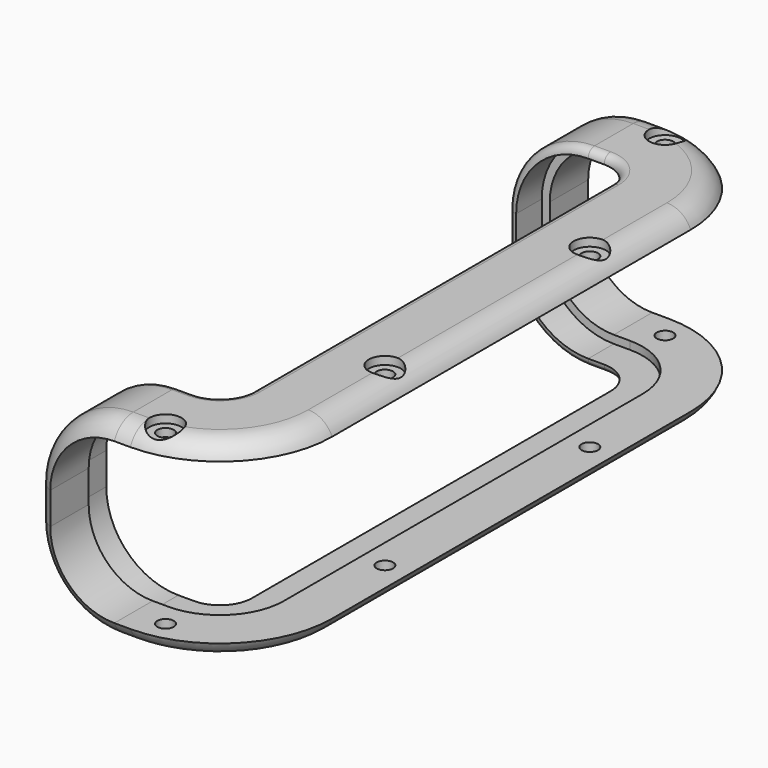
from build123d import *

# Parameters (mm, degrees)
F1_DEPTH      = 133.35
F2_R          = 12.7
F3_R          = 15.875
F4_R          = 22.225
F6_DEPTH      = 38.101
F8_DEPTH      = 6.35
F8_DEPTH_BACK = 107.95
F9_R          = 12.7
F10_T1_DEPTH  = 6.35
F10_T3_DEPTH  = 3.175
F10_T5_DEPTH  = 88.9
F10_T8_ANGLE  = 90
F10_T10_ANGLE = 90
F10_T12_ANGLE = 90
F10_T14_ANGLE = 90
F10_T16_ANGLE = 90
F10_T18_ANGLE = 90
F10_T20_ANGLE = 90
F10_T22_ANGLE = 90
F11_R         = 1.58749
F13_D         = 3.2639
F14_R         = 3.175
F15_DEPTH     = 1.5875


# Not quite as in the source:
# - a fillet or chamfer that OpenCascade refuses, or shapes differently, is made with other operations: its cross-section is extruded or revolved along the edge and cut away or added
# - a fillet or chamfer is up to 0.001 mm smaller than in the source, because OpenCascade refuses the exact size


with BuildPart() as f1:
    # F0 (on Front) → F1 (new body)
    with BuildSketch(Plane.XZ):
        Polygon((38.1, 0), (0, 0), (0, 31.75), (38.1, 31.75), (38.1, 34.925), (-3.175, 34.925), (-3.175, -3.175), (38.1, -3.175), align=None)
    extrude(amount=F1_DEPTH)

    # F2
    f2_edges = [f1.edges().sort_by_distance(p)[0] for p in [
        (0, -66.675, 0),
        (0, -66.675, 31.75),
    ]]
    fillet(f2_edges, radius=F2_R)

    # F3
    f3_edges = [f1.edges().sort_by_distance(p)[0] for p in [
        (-3.175, -66.675, -3.175),
        (-3.175, -66.675, 34.925),
    ]]
    fillet(f3_edges, radius=F3_R)

    # F4
    f4_edges = [f1.edges().sort_by_distance(p)[0] for p in [
        (38.1, -133.35, 33.3375),
        (38.1, -133.35, -1.5875),
        (38.1, 0, 33.3375),
        (38.1, 0, -1.5875),
    ]]
    fillet(f4_edges, radius=F4_R)

    # F5 (on face) → F6 (cut, through all)
    with BuildSketch(Plane.XY.offset(34.925)):
        with BuildLine():
            Line((-3.175, -117.475), (15.875, -117.475))
            ThreePointArc((15.875, -117.475), (20.3651280605, -115.6151280605), (22.225, -111.125))
            Line((22.225, -111.125), (22.225, -22.225))
            ThreePointArc((22.225, -22.225), (20.3651280605, -17.7348719395), (15.875, -15.875))
            Line((15.875, -15.875), (-3.175, -15.875))
            Line((-3.175, -15.875), (-3.175, -117.475))
        make_face()
    extrude(amount=-F6_DEPTH, mode=Mode.SUBTRACT)

    # F7 (on face) → F8 (cut, two sides)
    with BuildSketch(Plane(origin=(0, -117.475, 0), x_dir=(-1, 0, 0), z_dir=(0, 1, 0))) as f8_sk:
        with BuildLine():
            Line((-28.575, -1.5875), (-12.7, -1.5875))
            ThreePointArc((-12.7, -1.5875), (-2.5972118638, 2.5972118638), (1.5875, 12.7))
            Line((1.5875, 12.7), (1.5875, 19.05))
            ThreePointArc((1.5875, 19.05), (-2.5972118638, 29.1527881362), (-12.7, 33.3375))
            Line((-12.7, 33.3375), (-28.575, 33.3375))
            Line((-28.575, 33.3375), (-28.575, -1.5875))
        make_face()
    extrude(amount=-F8_DEPTH, mode=Mode.SUBTRACT)
    extrude(f8_sk.sketch, amount=F8_DEPTH_BACK, mode=Mode.SUBTRACT)

    # F9
    f9_edges = [f1.edges().sort_by_distance(p)[0] for p in [
        (28.575, -123.825, -0.79375),
        (28.575, -123.825, 32.54375),
        (28.575, -9.525, 32.54375),
        (28.575, -9.525, -0.79375),
    ]]
    fillet(f9_edges, radius=F9_R)

    # F10: fillet of radius 5.08 on 1 edges, made by hand

    # F10_s2 → F10_t1 (cut)
    with BuildSketch(Plane.XY.offset(12.7)):
        with BuildLine():
            ThreePointArc((0, -133.35), (-2.3071134838, -131.4805202921), (-3.175, -128.6407139607))
            Line((-3.175, -128.6407139607), (-3.175, -133.35))
            Line((-3.175, -133.35), (0, -133.35))
        make_face()
        with BuildLine():
            ThreePointArc((0, 0), (-2.3071134838, -1.8694797079), (-3.175, -4.7092860393))
            Line((-3.175, -4.7092860393), (-3.175, 0))
            Line((-3.175, 0), (0, 0))
        make_face()
    extrude(amount=F10_T1_DEPTH, mode=Mode.SUBTRACT)

    # F10_s4 → F10_t3 (cut)
    with BuildSketch(Plane.YZ.offset(12.7)):
        with BuildLine():
            ThreePointArc((-133.35, 31.75), (-131.4805202921, 34.0571134838), (-128.6407139607, 34.925))
            Line((-128.6407139607, 34.925), (-133.35, 34.925))
            Line((-133.35, 34.925), (-133.35, 31.75))
        make_face()
        with BuildLine():
            ThreePointArc((0, 31.75), (-1.8694797079, 34.0571134838), (-4.7092860393, 34.925))
            Line((-4.7092860393, 34.925), (0, 34.925))
            Line((0, 34.925), (0, 31.75))
        make_face()
        with BuildLine():
            ThreePointArc((0, 0), (-1.8694797079, -2.3071134838), (-4.7092860393, -3.175))
            Line((-4.7092860393, -3.175), (0, -3.175))
            Line((0, -3.175), (0, 0))
        make_face()
        with BuildLine():
            ThreePointArc((-133.35, 0), (-131.4805202921, -2.3071134838), (-128.6407139607, -3.175))
            Line((-128.6407139607, -3.175), (-133.35, -3.175))
            Line((-133.35, -3.175), (-133.35, 0))
        make_face()
    extrude(amount=F10_T3_DEPTH, mode=Mode.SUBTRACT)

    # F10_s6 → F10_t5 (cut)
    with BuildSketch(Plane.XZ.offset(22.225)):
        with BuildLine():
            ThreePointArc((33.3907139607, 34.925), (36.2305202921, 34.0571134838), (38.1, 31.75))
            Line((38.1, 31.75), (38.1, 34.925))
            Line((38.1, 34.925), (33.3907139607, 34.925))
        make_face()
        with BuildLine():
            ThreePointArc((38.1, 0), (36.2305202921, -2.3071134838), (33.3907139607, -3.175))
            Line((33.3907139607, -3.175), (38.1, -3.175))
            Line((38.1, -3.175), (38.1, 0))
        make_face()
    extrude(amount=F10_T5_DEPTH, mode=Mode.SUBTRACT)

    # F10_s7 → F10_t8 (revolve, cut)
    with BuildSketch(Plane.XY.offset(19.05)):
        with BuildLine():
            ThreePointArc((0, -133.35), (-2.3071134838, -131.4805202921), (-3.175, -128.6407139607))
            Line((-3.175, -128.6407139607), (-3.175, -133.35))
            Line((-3.175, -133.35), (0, -133.35))
        make_face()
    revolve(axis=Axis((12.7, -133.35, 19.05), (0, 1, 0)), revolution_arc=F10_T8_ANGLE, mode=Mode.SUBTRACT)

    # F10_s9 → F10_t10 (revolve, cut)
    with BuildSketch(Plane.XZ.offset(111.125)):
        with BuildLine():
            ThreePointArc((33.3907139607, 34.925), (36.2305202921, 34.0571134838), (38.1, 31.75))
            Line((38.1, 31.75), (38.1, 34.925))
            Line((38.1, 34.925), (33.3907139607, 34.925))
        make_face()
    revolve(axis=Axis((15.875, -111.125, 34.925), (0, 0, -1)), revolution_arc=F10_T10_ANGLE, mode=Mode.SUBTRACT)

    # F10_s11 → F10_t12 (revolve, cut)
    with BuildSketch(Plane.YZ.offset(15.875)):
        with BuildLine():
            ThreePointArc((-4.7092860393, 34.925), (-1.8694797079, 34.0571134838), (0, 31.75))
            Line((0, 31.75), (0, 34.925))
            Line((0, 34.925), (-4.7092860393, 34.925))
        make_face()
    revolve(axis=Axis((15.875, -22.225, 34.925), (0, 0, -1)), revolution_arc=F10_T12_ANGLE, mode=Mode.SUBTRACT)

    # F10_s13 → F10_t14 (revolve, cut)
    with BuildSketch(Plane.XY.offset(19.05)):
        with BuildLine():
            ThreePointArc((0, 0), (-2.3071134838, -1.8694797079), (-3.175, -4.7092860393))
            Line((-3.175, -4.7092860393), (-3.175, 0))
            Line((-3.175, 0), (0, 0))
        make_face()
    revolve(axis=Axis((12.7, 0, 19.05), (0, 1, 0)), revolution_arc=F10_T14_ANGLE, mode=Mode.SUBTRACT)

    # F10_s15 → F10_t16 (revolve, cut)
    with BuildSketch(Plane.YZ.offset(12.7)):
        with BuildLine():
            ThreePointArc((0, 0), (-1.8694797079, -2.3071134838), (-4.7092860393, -3.175))
            Line((-4.7092860393, -3.175), (0, -3.175))
            Line((0, -3.175), (0, 0))
        make_face()
    revolve(axis=Axis((12.7, 0, 12.7), (0, 1, 0)), revolution_arc=F10_T16_ANGLE, mode=Mode.SUBTRACT)

    # F10_s17 → F10_t18 (revolve, cut)
    with BuildSketch(Plane.YZ.offset(15.875)):
        with BuildLine():
            ThreePointArc((0, 0), (-1.8694797079, -2.3071134838), (-4.7092860393, -3.175))
            Line((-4.7092860393, -3.175), (0, -3.175))
            Line((0, -3.175), (0, 0))
        make_face()
    revolve(axis=Axis((15.875, -22.225, -3.175), (0, 0, -1)), revolution_arc=F10_T18_ANGLE, mode=Mode.SUBTRACT)

    # F10_s19 → F10_t20 (revolve, cut)
    with BuildSketch(Plane.XZ.offset(111.125)):
        with BuildLine():
            ThreePointArc((38.1, 0), (36.2305202921, -2.3071134838), (33.3907139607, -3.175))
            Line((33.3907139607, -3.175), (38.1, -3.175))
            Line((38.1, -3.175), (38.1, 0))
        make_face()
    revolve(axis=Axis((15.875, -111.125, -3.175), (0, 0, -1)), revolution_arc=F10_T20_ANGLE, mode=Mode.SUBTRACT)

    # F10_s21 → F10_t22 (revolve, cut)
    with BuildSketch(Plane.YZ.offset(12.7)):
        with BuildLine():
            ThreePointArc((-133.35, 0), (-131.4805202921, -2.3071134838), (-128.6407139607, -3.175))
            Line((-128.6407139607, -3.175), (-133.35, -3.175))
            Line((-133.35, -3.175), (-133.35, 0))
        make_face()
    revolve(axis=Axis((12.7, -133.35, 12.7), (0, 1, 0)), revolution_arc=F10_T22_ANGLE, mode=Mode.SUBTRACT)

    # F11 (radius 1.5875 in the source; OpenCascade refuses exactly that, so slightly less here)
    f11_edges = [f1.edges().sort_by_distance(p)[0] for p in [
        (1.47468, -117.475, 1.47468),
        (14.2875, -117.475, -3.175),
        (20.365128, -115.615128, -3.175),
        (22.225, -66.675, -3.175),
        (20.365128, -17.734872, -3.175),
        (14.2875, -15.875, -3.175),
        (14.2875, -15.875, 34.925),
        (1.47468, -15.875, 30.27532),
        (-3.175, -15.875, 15.875),
        (1.47468, -15.875, 1.47468),
        (14.2875, -117.475, 34.925),
        (-3.175, -117.475, 15.875),
        (1.47468, -117.475, 30.27532),
        (20.365128, -17.734872, 34.925),
        (22.225, -66.675, 34.925),
        (20.365128, -115.615128, 34.925),
    ]]
    fillet(f11_edges, radius=F11_R)

    # F13 (through all)
    with Locations(Plane.XY.offset(34.925)):
        with Locations((19.05, -4.7625), (33.3375, -41.275), (33.3375, -92.075), (19.05, -128.5875)):
            Hole(F13_D / 2)

    # F14 (on face) → F15 (cut)
    with BuildSketch(Plane.XY.offset(34.925)):
        with Locations((19.05, -4.7625)):
            Circle(F14_R)
        with Locations((33.3375, -41.275)):
            Circle(F14_R)
        with Locations((33.3375, -92.075)):
            Circle(F14_R)
        with Locations((19.05, -128.5875)):
            Circle(F14_R)
    extrude(amount=-F15_DEPTH, mode=Mode.SUBTRACT)


solid = f1.part
